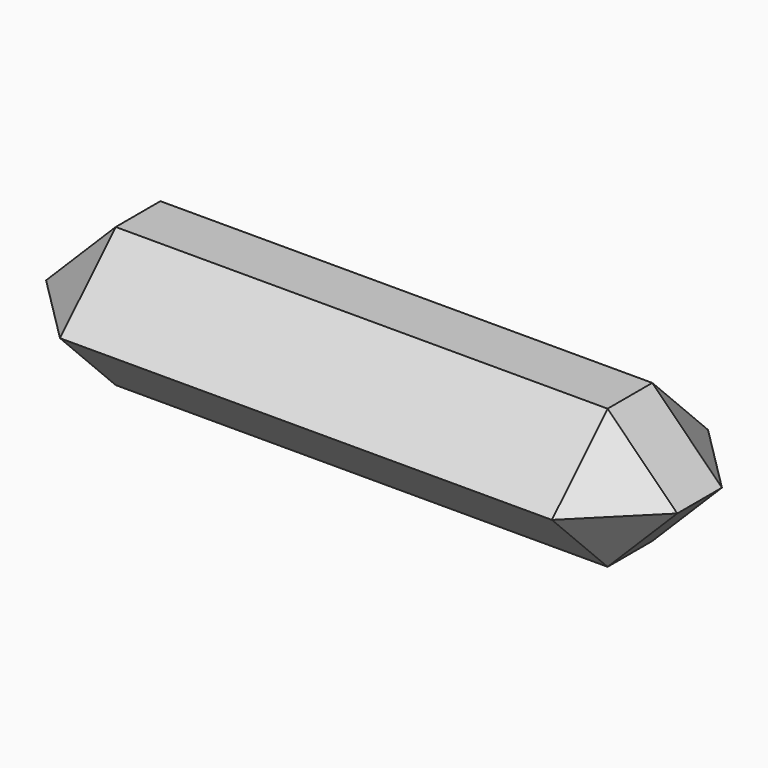
from build123d import *

# Parameters (mm, degrees)
F0_W     = 115.1367947459
F0_H     = 35.5919650756
F1_DEPTH = 25.4
F2_SIZE  = 12.69999


# Not quite as in the source:
# - a fillet or chamfer is up to 0.001 mm smaller than in the source, because OpenCascade refuses the exact size


with BuildPart() as f1:
    # F0 (on Top) → F1 (new body)
    with BuildSketch(Plane.XY):
        with Locations((0, 3.3258602489)):
            Rectangle(F0_W, F0_H)
    extrude(amount=F1_DEPTH)

    # F2 (size 12.7 in the source; OpenCascade refuses exactly that, so slightly less here)
    f2_edges = [f1.edges().sort_by_distance(p)[0] for p in [
        (0, -14.470122, 0),
        (57.568397, 21.121843, 12.7),
        (57.568397, -14.470122, 12.7),
        (57.568397, 3.32586, 0),
        (57.568397, 3.32586, 25.4),
        (0, 21.121843, 25.4),
        (0, 21.121843, 0),
        (-57.568397, 21.121843, 12.7),
        (0, -14.470122, 25.4),
        (-57.568397, 3.32586, 0),
        (-57.568397, -14.470122, 12.7),
        (-57.568397, 3.32586, 25.4),
    ]]
    chamfer(f2_edges, length=F2_SIZE)


solid = f1.part
